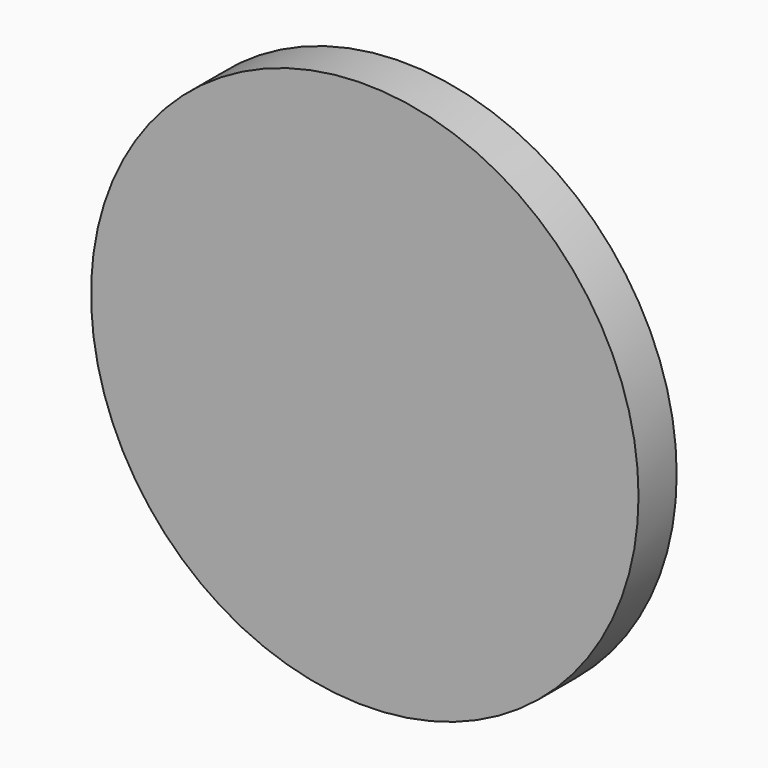
from build123d import *

# Parameters (mm, degrees)
F0_R         = 29.1605736942
F1_DEPTH     = 5.08
F2_TEXT_SIZE = 22.8904187679
F3_DEPTH     = 2.54


# Not quite as in the source:
# - Text() gives the source's letters only with a copy of the font that has no kerning and outlines rounded to 1/6400 em; it was checked with that copy


with BuildPart() as f1:
    # F0 (on Front) → F1 (new body)
    with BuildSketch(Plane.XZ):
        with Locations((-26.3669323176, -14.5472725853)):
            Circle(F0_R)
    extrude(amount=F1_DEPTH)

    # F2 (on Front) → F3 (cut)
    with BuildSketch(Plane.XZ):
        with Locations((-46.856155619, -22.0386842266)):
            Text('SSA', F2_TEXT_SIZE, font='Open Sans', font_style=FontStyle.BOLD, text_align=(TextAlign.LEFT, TextAlign.BOTTOM))
    extrude(amount=F3_DEPTH, mode=Mode.SUBTRACT)


solid = f1.part
